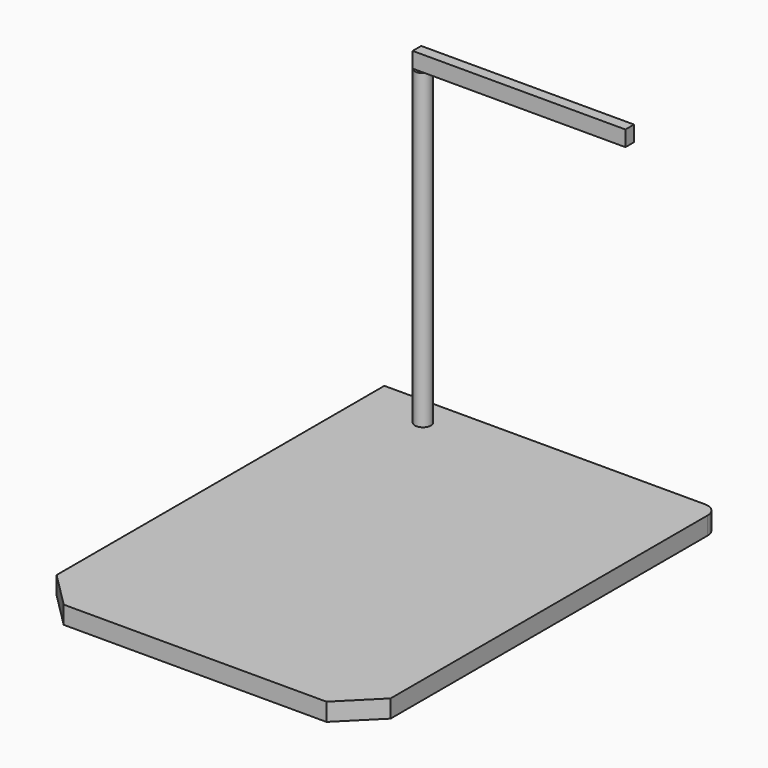
from build123d import *

# Parameters (mm, degrees)
F0_W     = 19.05
F0_H     = 25.4
F1_DEPTH = 1.016
F2_SIZE  = 2.032
F3_SIZE  = 2.032
F4_R     = 0.762
F5_R     = 0.4573869554
F6_DEPTH = 17.78
F9_DEPTH = 0.889


# Not quite as in the source:
# - the program builds the solid bodies; features that only make, move or delete a surface that nothing else refers to are left out


with BuildPart() as f1:
    # F0 (on Top) → F1 (new body)
    with BuildSketch(Plane.XY):
        with Locations((9.525, 12.7)):
            Rectangle(F0_W, F0_H)
    extrude(amount=F1_DEPTH)

    # F2
    f2_edges = [f1.edges().sort_by_distance(p)[0] for p in [
        (0, 0, 0.508),
    ]]
    chamfer(f2_edges, length=F2_SIZE)

    # F3
    f3_edges = [f1.edges().sort_by_distance(p)[0] for p in [
        (19.05, 0, 0.508),
    ]]
    chamfer(f3_edges, length=F3_SIZE)

    # F4
    f4_edges = [f1.edges().sort_by_distance(p)[0] for p in [
        (19.05, 25.4, 0.508),
    ]]
    fillet(f4_edges, radius=F4_R)

    # F5 (on face) → F6 (join)
    with BuildSketch(Plane.XY.offset(1.016)):
        with Locations((3.5583837889, 23.701650244)):
            Circle(F5_R)
    extrude(amount=F6_DEPTH)

    # F8 (on face) → F9 (join)
    with BuildSketch(Plane.XY.offset(18.796)):
        with BuildLine():
            ThreePointArc((4.0157707443, 23.701650244), (3.9885840141, 23.5463099941), (3.9102557402, 23.4094363551))
            Line((3.9102557402, 23.4094363551), (15.3415361419, 23.4094363551))
            Line((15.3415361419, 23.4094363551), (15.3415361419, 24.0212995559))
            Line((15.3415361419, 24.0212995559), (3.8855338223, 24.0212995559))
            ThreePointArc((3.8855338223, 24.0212995559), (3.9819619899, 23.8742316295), (4.0157707443, 23.701650244))
        make_face()
        with BuildLine():
            Line((3.2065118376, 23.9938641329), (3.2065118376, 23.4094363551))
            Line((3.2065118376, 23.4094363551), (3.9102557402, 23.4094363551))
            ThreePointArc((3.9102557402, 23.4094363551), (3.9885840141, 23.5463099941), (4.0157707443, 23.701650244))
            ThreePointArc((4.0157707443, 23.701650244), (3.9819619899, 23.8742316295), (3.8855338223, 24.0212995559))
            Line((3.8855338223, 24.0212995559), (3.2312337555, 24.0212995559))
            ThreePointArc((3.2312337555, 24.0212995559), (3.2185957822, 24.0078314607), (3.2065118376, 23.9938641329))
        make_face()
    extrude(amount=F9_DEPTH)


solid = f1.part
